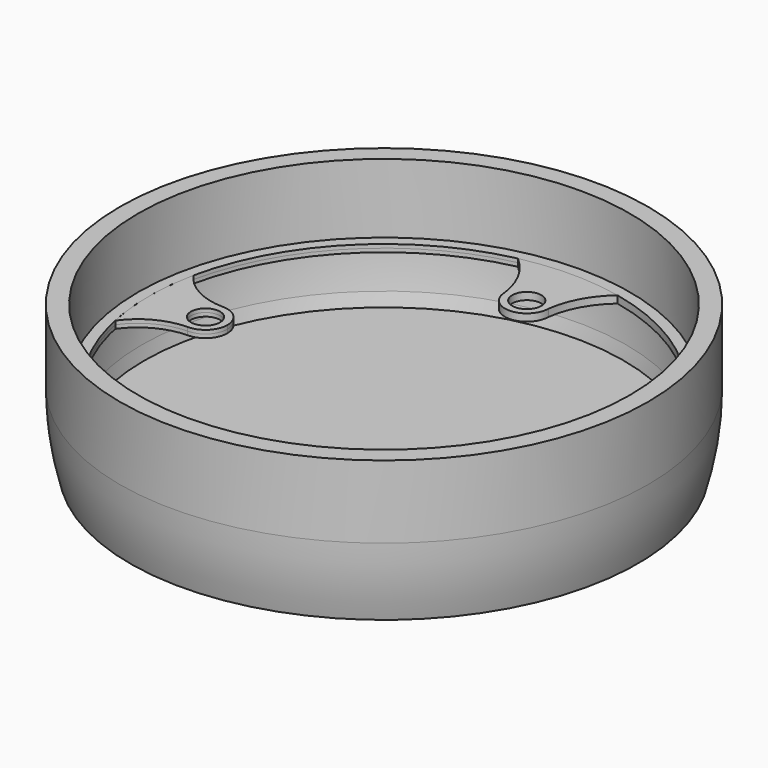
from build123d import *

# Parameters (mm, degrees)
F0_R     = 4
F1_DEPTH = 1
F0_R_2   = 67.5
F3_DEPTH = 1


with BuildPart() as f1:
    # F0 (on Top) → F1 (new body, symmetric)
    with BuildSketch(Plane.XY):
        with BuildLine():
            ThreePointArc((63.085609693, -13.4333856366), (64.1454278386, -6.7538202079), (64.5, 0))
            ThreePointArc((64.5, 0), (64.1454278386, 6.7538202079), (63.085609693, 13.4333856366))
            ThreePointArc((63.085609693, 13.4333856366), (56.974835778, 8.034166581), (49.0784312352, 5.9994873565))
            ThreePointArc((49.0784312352, 5.9994873565), (53.2702802842, 4.2148198413), (55, 0))
            ThreePointArc((55, 0), (53.2702802842, -4.2148198413), (49.0784312352, -5.9994873565))
            ThreePointArc((49.0784312352, -5.9994873565), (56.974835778, -8.034166581), (63.085609693, -13.4333856366))
        make_face()
        with BuildLine():
            ThreePointArc((55, 0), (53.2702802842, 4.2148198413), (49.0784312352, 5.9994873565))
            ThreePointArc((49.0784312352, 5.9994873565), (43, 0), (49.0784312352, -5.9994873565))
            ThreePointArc((49.0784312352, -5.9994873565), (53.2702802842, -4.2148198413), (55, 0))
        make_face()
        with Locations((49, 0)):
            Circle(F0_R, mode=Mode.SUBTRACT)
    extrude(amount=F1_DEPTH, both=True)


with BuildPart() as f1b:
    # F0 (on Top) → F1, piece 2 (new body, symmetric)
    with BuildSketch(Plane.XY):
        with BuildLine():
            ThreePointArc((5.9988880077, 48.8844895219), (8.515751779, 56.6748662417), (13.671329053, 63.034472806))
            ThreePointArc((13.671329053, 63.034472806), (0, 64.5), (-13.671329053, 63.034472806))
            ThreePointArc((-13.671329053, 63.034472806), (-8.515751779, 56.6748662417), (-5.9988880077, 48.8844895219))
            ThreePointArc((-5.9988880077, 48.8844895219), (-0.0577579152, 54.9997219955), (6, 49))
            ThreePointArc((6, 49), (5.9997219955, 48.9422420848), (5.9988880077, 48.8844895219))
        make_face()
        with BuildLine():
            ThreePointArc((-5.9988880077, 48.8844895219), (0, 43), (5.9988880077, 48.8844895219))
            ThreePointArc((5.9988880077, 48.8844895219), (5.9997219955, 48.9422420848), (6, 49))
            ThreePointArc((6, 49), (-0.0577579152, 54.9997219955), (-5.9988880077, 48.8844895219))
        make_face()
        with Locations((0, 49)):
            Circle(F0_R, mode=Mode.SUBTRACT)
    extrude(amount=F1_DEPTH, both=True)


with BuildPart() as f1c:
    # F0 (on Top) → F1, piece 3 (new body, symmetric)
    with BuildSketch(Plane.XY):
        with BuildLine():
            ThreePointArc((-13.671329053, -63.034472806), (0, -64.5), (13.671329053, -63.034472806))
            ThreePointArc((13.671329053, -63.034472806), (8.515751779, -56.6748662417), (5.9988880077, -48.8844895219))
            ThreePointArc((5.9988880077, -48.8844895219), (5.9997219955, -48.9422420848), (6, -49))
            ThreePointArc((6, -49), (-0.0577579152, -54.9997219955), (-5.9988880077, -48.8844895219))
            ThreePointArc((-5.9988880077, -48.8844895219), (-8.515751779, -56.6748662417), (-13.671329053, -63.034472806))
        make_face()
        with BuildLine():
            ThreePointArc((6, -49), (5.9997219955, -48.9422420848), (5.9988880077, -48.8844895219))
            ThreePointArc((5.9988880077, -48.8844895219), (0, -43), (-5.9988880077, -48.8844895219))
            ThreePointArc((-5.9988880077, -48.8844895219), (-0.0577579152, -54.9997219955), (6, -49))
        make_face()
        with Locations((0, -49)):
            Circle(F0_R, mode=Mode.SUBTRACT)
    extrude(amount=F1_DEPTH, both=True)


with BuildPart() as f1d:
    # F0 (on Top) → F1, piece 4 (new body, symmetric)
    with BuildSketch(Plane.XY):
        with BuildLine():
            ThreePointArc((-49.0784312352, 5.9994873565), (-56.974835778, 8.034166581), (-63.085609693, 13.4333856366))
            ThreePointArc((-63.085609693, 13.4333856366), (-64.5, 0), (-63.085609693, -13.4333856366))
            ThreePointArc((-63.085609693, -13.4333856366), (-56.974835778, -8.034166581), (-49.0784312352, -5.9994873565))
            ThreePointArc((-49.0784312352, -5.9994873565), (-55, 0), (-49.0784312352, 5.9994873565))
        make_face()
        with BuildLine():
            ThreePointArc((-43, 0), (-44.7851801587, 4.2702802842), (-49.0784312352, 5.9994873565))
            ThreePointArc((-49.0784312352, 5.9994873565), (-55, 0), (-49.0784312352, -5.9994873565))
            ThreePointArc((-49.0784312352, -5.9994873565), (-44.7851801587, -4.2702802842), (-43, 0))
        make_face()
        with Locations((-49, 0)):
            Circle(F0_R, mode=Mode.SUBTRACT)
    extrude(amount=F1_DEPTH, both=True)


with BuildPart() as f3:
    # F0 (on Top) → F3 (new body, symmetric)
    with BuildSketch(Plane.XY):
        Circle(F0_R_2)
        with BuildLine():
            ThreePointArc((63.085609693, 13.4333856366), (64.1454278386, 6.7538202079), (64.5, 0))
            ThreePointArc((64.5, 0), (64.1454278386, -6.7538202079), (63.085609693, -13.4333856366))
            ThreePointArc((63.085609693, -13.4333856366), (45.6943527529, -45.5222596813), (13.671329053, -63.034472806))
            ThreePointArc((13.671329053, -63.034472806), (0, -64.5), (-13.671329053, -63.034472806))
            ThreePointArc((-13.671329053, -63.034472806), (-45.6943527529, -45.5222596813), (-63.085609693, -13.4333856366))
            ThreePointArc((-63.085609693, -13.4333856366), (-64.5, 0), (-63.085609693, 13.4333856366))
            ThreePointArc((-63.085609693, 13.4333856366), (-45.6943527529, 45.5222596813), (-13.671329053, 63.034472806))
            ThreePointArc((-13.671329053, 63.034472806), (0, 64.5), (13.671329053, 63.034472806))
            ThreePointArc((13.671329053, 63.034472806), (45.6943527529, 45.5222596813), (63.085609693, 13.4333856366))
        make_face(mode=Mode.SUBTRACT)
    extrude(amount=F3_DEPTH, both=True)

    # F2 (on Front) → F4 (revolve)
    with BuildSketch(Plane.XZ):
        with BuildLine():
            Line((0, -15), (-65.8122329054, -15))
            ThreePointArc((-65.8122329054, -15), (-66.1917705208, -13.2249580461), (-66.5234419851, -11.4403525492))
            ThreePointArc((-66.5234419851, -11.4403525492), (-67.215928307, -6.1861928378), (-67.4940807973, -0.893900067))
            ThreePointArc((-67.4940807973, -0.893900067), (-67.4985201831, -0.4469598323), (-67.5, 0))
            Line((-67.5, 0), (-67.5, 20))
            Line((-67.5, 20), (-72.5, 20))
            Line((-72.5, 20), (-72.5, 0))
            ThreePointArc((-72.5, 0), (-71.7932550835, -10.0984416873), (-69.6867993238, -20))
            Line((-69.6867993238, -20), (0, -20))
            Line((0, -20), (0, -15))
        make_face()
    revolve(axis=Axis((0, 0, 7.5), (0, 0, -1)))


solid = Compound([f1.part, f1b.part, f1c.part, f1d.part, f3.part])
